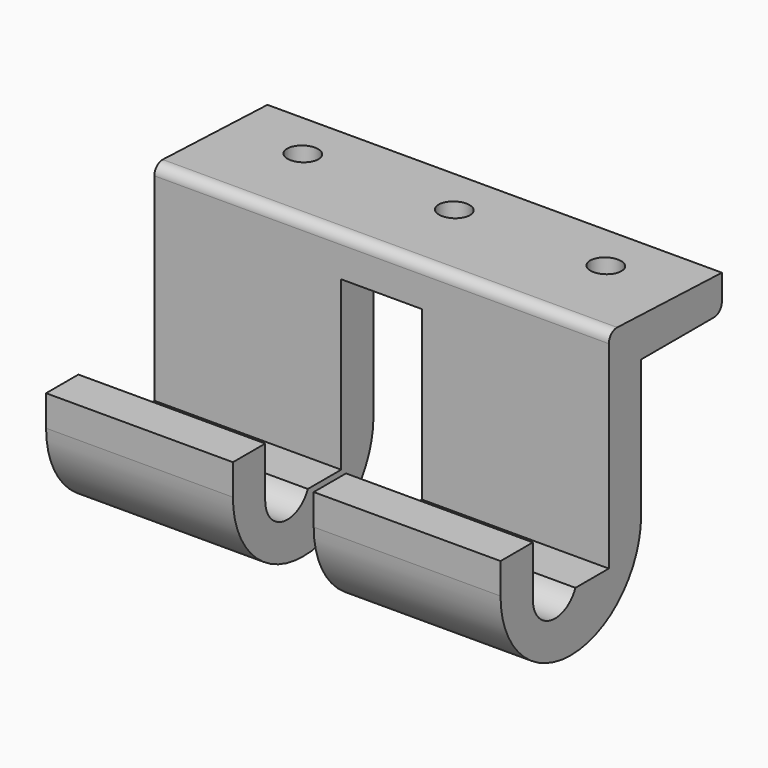
from build123d import *

# Parameters (mm, degrees)
F0_W        = 45
F0_H        = 26.25
F1_DEPTH    = 17.4
F2_W        = 45
F2_H        = 4
F3_DEPTH    = 10
F5_DEPTH    = 45
F7_D        = 3
F8_T1_DEPTH = 112.5981529113
F9_W        = 8
F9_H        = 22.25
F9_H_2      = 1.1180170857
F10_DEPTH   = 21.5
F11_R       = 8.69999
F12_R       = 1


# Not quite as in the source:
# - a fillet or chamfer that OpenCascade refuses, or shapes differently, is made with other operations: its cross-section is extruded or revolved along the edge and cut away or added
# - a fillet or chamfer is up to 0.001 mm smaller than in the source, because OpenCascade refuses the exact size


with BuildPart() as f1:
    # F0 (on Front) → F1 (new body)
    with BuildSketch(Plane.XZ):
        Rectangle(F0_W, F0_H)
    extrude(amount=F1_DEPTH)

    # F2 (on face) → F3 (join)
    with BuildSketch(Plane(origin=(0, 0, 0), x_dir=(-1, 0, 0), z_dir=(0, 1, 0))):
        with Locations((0, 11.125)):
            Rectangle(F2_W, F2_H)
    extrude(amount=F3_DEPTH)

    # F4 (on face) → F5 (cut)
    with BuildSketch(Plane.YZ.offset(22.5)):
        with BuildLine():
            Line((-13.4, -1.375), (-13.4, -6.375))
            ThreePointArc((-13.4, -6.375), (-11.2118515201, -9.0669923606), (-8.1295833678, -7.475))
            Line((-8.1295833678, -7.475), (-4.5024615599, -7.475))
            Line((-4.5024615599, -7.475), (-4, -7.475))
            Line((-4, -7.475), (-4, 13.125))
            Line((-4, 13.125), (-17.4, 13.125))
            Line((-17.4, 13.125), (-17.4, -1.375))
            Line((-17.4, -1.375), (-13.4, -1.375))
        make_face()
    extrude(amount=-F5_DEPTH, mode=Mode.SUBTRACT)

    # F7 (through all)
    with Locations(Plane(origin=(0, 0, 9.125), x_dir=(1, 0, 0), z_dir=(0, 0, -1))):
        with Locations((-15, -5), (0, -5), (15, -5)):
            Hole(F7_D / 2)

    # F8: chamfer of 13 x 0.5 on 1 edges, made by hand

    # F8_s2 → F8_t1 (cut)
    with BuildSketch(Plane.YZ.offset(-56.2990764557)):
        Polygon((-3, 13.125), (10, 12.625), (10, 13.125), align=None)
    extrude(amount=F8_T1_DEPTH, mode=Mode.SUBTRACT)

    # F9 (on face) → F10 (cut)
    with BuildSketch(Plane(origin=(0, 0, 0), x_dir=(-1, 0, 0), z_dir=(0, 1, 0))):
        with Locations((0, -2)):
            Rectangle(F9_W, F9_H)
        with Locations((0, -13.6840085428)):
            Rectangle(F9_W, F9_H_2)
    extrude(amount=-F10_DEPTH, mode=Mode.SUBTRACT)

    # F11 (radius 8.7 in the source; OpenCascade refuses exactly that, so slightly less here)
    f11_edges = [f1.edges().sort_by_distance(p)[0] for p in [
        (-13.25, -17.4, -13.125),
        (-13.25, 0, -13.125),
        (13.25, -17.4, -13.125),
        (13.25, 0, -13.125),
    ]]
    fillet(f11_edges, radius=F11_R)

    # F12
    f12_edges = [f1.edges().sort_by_distance(p)[0] for p in [
        (0, 10, 9.125),
        (0, -4, 13.125),
    ]]
    fillet(f12_edges, radius=F12_R)


solid = f1.part
